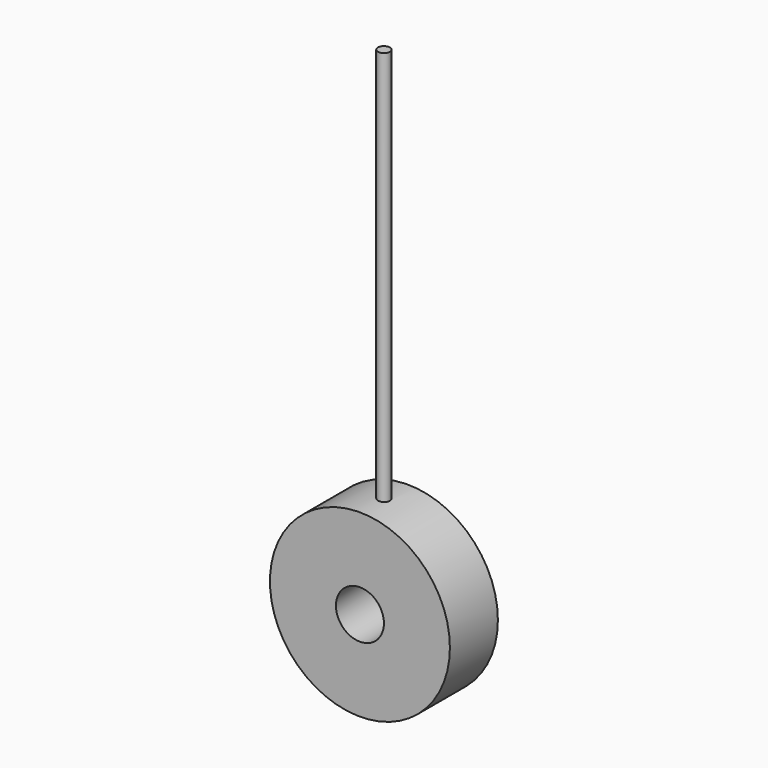
from build123d import *

# Parameters (mm, degrees)
F3_R     = 19.05
F4_DEPTH = 6.35
F5_R     = 1.27
F6_DEPTH = 102.6929366
F7_R     = 5.08
F8_DEPTH = 12.701
F9_DEPTH = 109.0429366


# Not quite as in the source:
# - the program builds the solid bodies; features that only make, move or delete a surface that nothing else refers to are left out


with BuildPart() as f4:
    # F3 (on face) → F4 (new body, symmetric)
    with BuildSketch(Plane.XZ):
        Circle(F3_R)
    extrude(amount=F4_DEPTH, both=True)


with BuildPart() as f6:
    # F5 (on Top) → F6 (new body)
    with BuildSketch(Plane.XY):
        Circle(F5_R)
    extrude(amount=F6_DEPTH)


with BuildPart() as f8_tool:
    # F7 (on face) → F8 (new body, through all)
    with BuildSketch(Plane.XZ.offset(6.35)):
        Circle(F7_R)
    extrude(amount=-F8_DEPTH)


with BuildPart() as f4_1:
    add(f4.part)

    # F8: cut by f8_tool
    add(f8_tool.part, mode=Mode.SUBTRACT)

    # F5 (on Top) → F9 (cut)
    with BuildSketch(Plane.XY):
        Circle(F5_R)
    extrude(amount=F9_DEPTH, mode=Mode.SUBTRACT)


with BuildPart() as f6_1:
    add(f6.part)

    # F8: cut by f8_tool
    add(f8_tool.part, mode=Mode.SUBTRACT)


solid = Compound([f4_1.part, f6_1.part])
